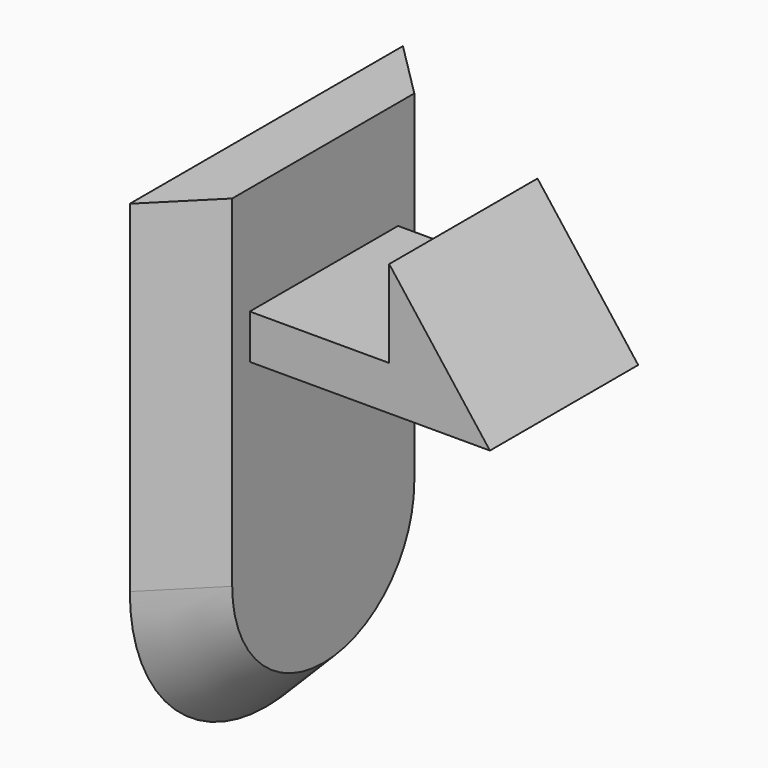
from build123d import *

# Parameters (mm, degrees)
F0_W     = 12
F0_H     = 18
F1_DEPTH = 2
F3_R     = 5.99999
F4_SIZE  = 1.99999
F5_W     = 6.5143028369
F5_H     = 4.6212589368
F6_DEPTH = 10
F7_W     = 4.9025638513
F7_H     = 3.0622794293
F8_DEPTH = 25


# Not quite as in the source:
# - a fillet or chamfer is up to 0.001 mm smaller than in the source, because OpenCascade refuses the exact size


with BuildPart() as f1:
    # F0 (on Right) → F1 (new body)
    with BuildSketch(Plane.YZ):
        Rectangle(F0_W, F0_H)
    extrude(amount=F1_DEPTH)

    # F3 (radius 6 in the source; OpenCascade refuses exactly that, so slightly less here)
    f3_edges = [f1.edges().sort_by_distance(p)[0] for p in [
        (1, 6, -9),
        (1, -6, -9),
    ]]
    fillet(f3_edges, radius=F3_R)

    # F4 (size 2 in the source; OpenCascade refuses exactly that, so slightly less here)
    f4_edges = [f1.edges().sort_by_distance(p)[0] for p in [
        (2, 4.242644, -7.242644),
        (2, -6, 2.999995),
    ]]
    chamfer(f4_edges, length=F4_SIZE)

    # F5 (on face) → F6 (join)
    with BuildSketch(Plane.YZ.offset(2)):
        with Locations((0.0278381212, 5.9414044954)):
            Rectangle(F5_W, F5_H)
    extrude(amount=F6_DEPTH)

    # F7 (on face) → F8 (cut)
    with BuildSketch(Plane.XZ.offset(3.2293132972)):
        Polygon((6.9025638513, 9.0315220878), (6.9025638513, 8.2520339638), (10.911365971, 3.0183200724), (13.6395776644, 3.0183200724), (12.8879277036, 9.0315220878), align=None)
        with Locations((4.4512819257, 6.7208942492)):
            Rectangle(F7_W, F7_H)
    extrude(amount=-F8_DEPTH, mode=Mode.SUBTRACT)


solid = f1.part
